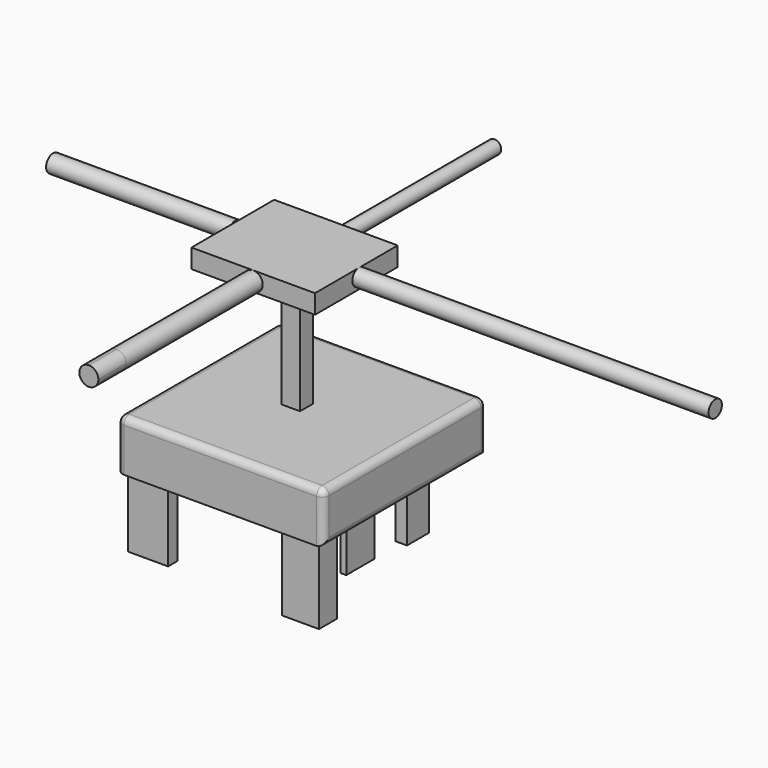
from build123d import *
from build123d import SkipClean  # not in build123d's __all__

# Parameters (mm, degrees)
F0_W          = 151.5855640173
F0_H          = 149.6286615729
F1_DEPTH      = 11.684
F2_DEPTH      = 25.4
F3_W          = 4.1966233402
F3_H          = 25.7666455582
F3_W_2        = 24.8086545616
F3_H_2        = 24.7343285009
F3_W_3        = 8.3932466805
F3_H_3        = 20.2822238207
F3_W_4        = 29.5776501298
F3_H_4        = 8.4610134363
F5_DEPTH      = 25.4
F6_DEPTH      = 25.4
F8_W          = 13.618723955
F8_H          = 11.8162455037
F9_DEPTH      = 88.646
F10_W         = 90.7247327268
F10_H         = 75.9043544531
F11_DEPTH     = 13.97
F13_DEPTH     = 25.4
F14_DEPTH     = 125.476
F16_DEPTH     = 25.4
F17_R         = 4.969033059
F18_DEPTH     = 117.348
F20_DEPTH     = 87.376
F21_R         = 6.1087740457
F22_DEPTH     = 25.4
F23_DEPTH     = 25.4
F24_DEPTH     = 25.4
F25_R         = 5.08
F26_T1_DEPTH  = 44.704
F26_S5_W      = 5.08
F26_S5_H      = 5.08
F26_T6_DEPTH  = 5.08
F26_S11_W     = 5.08
F26_S11_H     = 5.08
F26_T12_DEPTH = 5.08
F27_W         = 27.1943286061
F27_H         = 16.5108405054
F28_DEPTH     = 61.722
F29_DEPTH     = 25.4
F30_DEPTH     = 160.02
F31_DEPTH     = 46.482


# Not quite as in the source:
# - a fillet or chamfer that OpenCascade refuses, or shapes differently, is made with other operations: its cross-section is extruded or revolved along the edge and cut away or added
# - after a boolean that leaves OpenCascade's solid faulty, fix() repairs it
# - a feature names something its author has since deleted; it is built from what else it names


with BuildPart() as f1:
    # F0 (on Top) → F1 (new body)
    with BuildSketch(Plane.XY):
        with Locations((1.5608146787, -0.5317740142)):
            Rectangle(F0_W, F0_H)
    extrude(amount=F1_DEPTH)

    # F2 (add): a face of the model
    f2_faces = [f1.faces().sort_by_distance(p)[0] for p in [
        (1.5608146787, -0.5317740142, 0),
    ]]
    extrude(f2_faces, amount=F2_DEPTH)

    # F3 (on face) → F5 (join)
    with BuildSketch(Plane(origin=(0, 0, -25.4), x_dir=(1, 0, 0), z_dir=(0, 0, -1))):
        with Locations((45.1576719061, 3.9362064563)):
            Rectangle(F3_W, F3_H)
        with Locations((-27.7178613469, -21.3142805733)):
            Rectangle(F3_W_2, F3_H_2)
        with Locations((47.2559835762, -43.8225567341)):
            Rectangle(F3_W_3, F3_H_3)
        with Locations((-54.0488772094, 67.9751783609)):
            Rectangle(F3_W_4, F3_H_4)
    extrude(amount=F5_DEPTH)

    # F6 (add): faces of the model
    f6_faces = [f1.faces().sort_by_distance(p)[0] for p in [
        (-54.0488772094, -67.9751783609, -50.8),
        (-27.7178613469, 21.3142805733, -50.8),
        (45.1576719061, -3.9362064563, -50.8),
        (47.2559835762, 43.8225567341, -50.8),
    ]]
    extrude(f6_faces, amount=F6_DEPTH)

    # F8 (on face) → F9 (join)
    with BuildSketch(Plane.XY.offset(11.684)):
        with Locations((-1.9266440067, -0.4005506635)):
            Rectangle(F8_W, F8_H)
    extrude(amount=F9_DEPTH)

    # F10 (on face) → F11 (join)
    with BuildSketch(Plane.XY.offset(100.33)):
        with Locations((-2.2270549089, -2.4033039808)):
            Rectangle(F10_W, F10_H)
    extrude(amount=F11_DEPTH)

    # F12 (on face) → F13 (join)
    with BuildSketch(Plane.XZ.offset(40.3554812074)):
        with BuildLine():
            ThreePointArc((-2.2270549227, 100.33), (2.7120859528, 102.3758591285), (4.7579450911, 107.315))
            ThreePointArc((4.7579450911, 107.315), (2.712085945, 112.2541408793), (-2.227054945, 114.3))
            ThreePointArc((-2.227054945, 114.3), (-9.2120549089, 107.3149999888), (-2.2270549227, 100.33))
        make_face()
    extrude(amount=F13_DEPTH)

    # F14 (add): a face of the model
    f14_faces = [f1.faces().sort_by_distance(p)[0] for p in [
        (-2.2270549089, -65.7554812074, 107.315),
    ]]
    with SkipClean():  # cleaning this boolean's faces spoils the solid; the shape is the same uncleaned
        extrude(f14_faces, amount=F14_DEPTH)

    # F15 (on face) → F16 (join)
    with BuildSketch(Plane.YZ.offset(43.1353114545)):
        with BuildLine():
            Line((-1.1355586467, 114.3), (1.1355586467, 114.3))
            ThreePointArc((1.1355586467, 114.3), (0, 114.4064722454), (-1.1355586467, 114.3))
        make_face()
        with BuildLine():
            ThreePointArc((-1.1355586467, 114.3), (-3.8974510358, 103.5937641266), (6.1087740457, 108.2976981997))
            ThreePointArc((6.1087740457, 108.2976981997), (4.7039340732, 112.1951492356), (1.1355586467, 114.3))
            Line((1.1355586467, 114.3), (-1.1355586467, 114.3))
        make_face()
    extrude(amount=F16_DEPTH)

    add(f1.part.fix(), mode=Mode.REPLACE)

    # F17 (on face) → F18 (join)
    with BuildSketch(Plane(origin=(0, 35.5488732457, 0), x_dir=(-1, 0, 0), z_dir=(0, 1, 0))):
        with Locations((0, 105.8959811926)):
            Circle(F17_R)
    extrude(amount=F18_DEPTH)

    # F19 (on face) → F20 (join)
    with BuildSketch(Plane(origin=(-47.5894212723, 0, 0), x_dir=(0, -1, 0), z_dir=(-1, 0, 0))):
        with BuildLine():
            Line((-3.5482673546, 114.3), (3.5482673546, 114.3))
            ThreePointArc((3.5482673546, 114.3), (0, 115.3617326707), (-3.5482673546, 114.3))
        make_face()
        with BuildLine():
            ThreePointArc((-3.5482673546, 114.3), (-3.0667012813, 103.2161631583), (6.4599488467, 108.901783824))
            ThreePointArc((6.4599488467, 108.901783824), (5.6856206657, 111.9684851053), (3.5482673546, 114.3))
            Line((3.5482673546, 114.3), (-3.5482673546, 114.3))
        make_face()
    extrude(amount=F20_DEPTH)

    # F21 (on face) → F22 (join)
    with BuildSketch(Plane.YZ.offset(68.5353114545)):
        with Locations((0, 108.2976981997)):
            Circle(F21_R)
    extrude(amount=F22_DEPTH)

    # F23 (add): faces of the model
    f23_faces = [f1.faces().sort_by_distance(p)[0] for p in [
        (0, 152.8968732457, 105.8959811926),
        (-2.2270549089, -191.2314812074, 107.315),
    ]]
    extrude(f23_faces, amount=F23_DEPTH, dir=(0, 1, 0))

    # F24 (add): a face of the model
    f24_faces = [f1.faces().sort_by_distance(p)[0] for p in [
        (93.9353114545, 0, 108.2976981997),
    ]]
    extrude(f24_faces, amount=F24_DEPTH)

    # F25
    f25_edges = [f1.edges().sort_by_distance(p)[0] for p in [
        (77.353597, -0.531774, 11.684),
        (1.560815, -75.346105, 11.684),
        (-74.231967, -0.531774, 11.684),
        (1.560815, 74.282557, 11.684),
        (77.353597, -75.346105, -6.858),
        (77.353597, 74.282557, -6.858),
        (77.353597, -0.531774, -25.4),
    ]]
    fillet(f25_edges, radius=F25_R)

    # F26: fillet of radius 5.08 on 2 edges, made by hand

    # F26_s2 → F26_t1 (cut)
    with BuildSketch(Plane.XY.offset(-38.1)):
        with BuildLine():
            ThreePointArc((-69.15196733, -75.3461048007), (-72.7440697784, -73.8582072491), (-74.23196733, -70.2661048007))
            Line((-74.23196733, -70.2661048007), (-74.23196733, -75.3461048007))
            Line((-74.23196733, -75.3461048007), (-69.15196733, -75.3461048007))
        make_face()
        with BuildLine():
            ThreePointArc((-69.15196733, 74.2825567722), (-72.7440697784, 72.7946592207), (-74.23196733, 69.2025567722))
            Line((-74.23196733, 69.2025567722), (-74.23196733, 74.2825567722))
            Line((-74.23196733, 74.2825567722), (-69.15196733, 74.2825567722))
        make_face()
    extrude(amount=F26_T1_DEPTH, mode=Mode.SUBTRACT)


with BuildPart() as f26_tool4:
    # F26_s5 → F26_t6 (new body)
    with BuildSketch(Plane.XZ.offset(-69.2025567722)):
        with Locations((-71.69196733, 9.144)):
            Rectangle(F26_S5_W, F26_S5_H)
    extrude(amount=-F26_T6_DEPTH)

    # F26_s7 → F26_t8 (revolve, cut)
    with BuildSketch(Plane(origin=(-69.15196733, 69.2025567722, 6.604), x_dir=(0.7071067812, 0, -0.7071067812), z_dir=(0.7071067812, 0, 0.7071067812))):
        with BuildLine():
            ThreePointArc((0, -5.08), (5.08, 0), (0, 5.08))
            Line((0, 5.08), (0, -5.08))
        make_face()
    revolve(axis=Axis((-69.15196733, 69.2025567722, 6.604), (0, 1, 0)), mode=Mode.SUBTRACT)


with BuildPart() as f1_1:
    add(f1.part, clean=False)

    # F26_t3: cut F26_tool4
    add(f26_tool4.part, mode=Mode.SUBTRACT)


with BuildPart() as f26_tool10:
    # F26_s11 → F26_t12 (new body)
    with BuildSketch(Plane.XZ.offset(70.2661048007)):
        with Locations((-71.69196733, 9.144)):
            Rectangle(F26_S11_W, F26_S11_H)
    extrude(amount=F26_T12_DEPTH)

    # F26_s13 → F26_t14 (revolve, cut)
    with BuildSketch(Plane(origin=(-69.15196733, -70.2661048007, 6.604), x_dir=(0.7071067812, 0, -0.7071067812), z_dir=(-0.7071067812, 0, -0.7071067812))):
        with BuildLine():
            ThreePointArc((0, -5.08), (5.08, 0), (0, 5.08))
            Line((0, 5.08), (0, -5.08))
        make_face()
    revolve(axis=Axis((-69.15196733, -70.2661048007, 6.604), (0, -1, 0)), mode=Mode.SUBTRACT)


with BuildPart() as f1_2:
    add(f1_1.part, clean=False)

    # F26_t9: cut F26_tool10
    add(f26_tool10.part, mode=Mode.SUBTRACT)

    # F27 (on face) → F28 (join)
    with BuildSketch(Plane(origin=(0, 0, -25.4), x_dir=(1, 0, 0), z_dir=(0, 0, -1))):
        with Locations((50.2156950533, 54.3001759797)):
            Rectangle(F27_W, F27_H)
    extrude(amount=F28_DEPTH)

    # F29 (add): a face of the model
    f29_faces = [f1_2.faces().sort_by_distance(p)[0] for p in [
        (119.3353114545, 0, 108.2976981997),
    ]]
    extrude(f29_faces, amount=F29_DEPTH)

    # F30 (add): a face of the model
    f30_faces = [f1_2.faces().sort_by_distance(p)[0] for p in [
        (144.7353114545, 0, 108.2976981997),
    ]]
    extrude(f30_faces, amount=F30_DEPTH)

    # F31 (add): a face of the model
    f31_faces = [f1_2.faces().sort_by_distance(p)[0] for p in [
        (-134.9654212723, 0, 108.901783824),
    ]]
    extrude(f31_faces, amount=F31_DEPTH)


solid = f1_2.part
